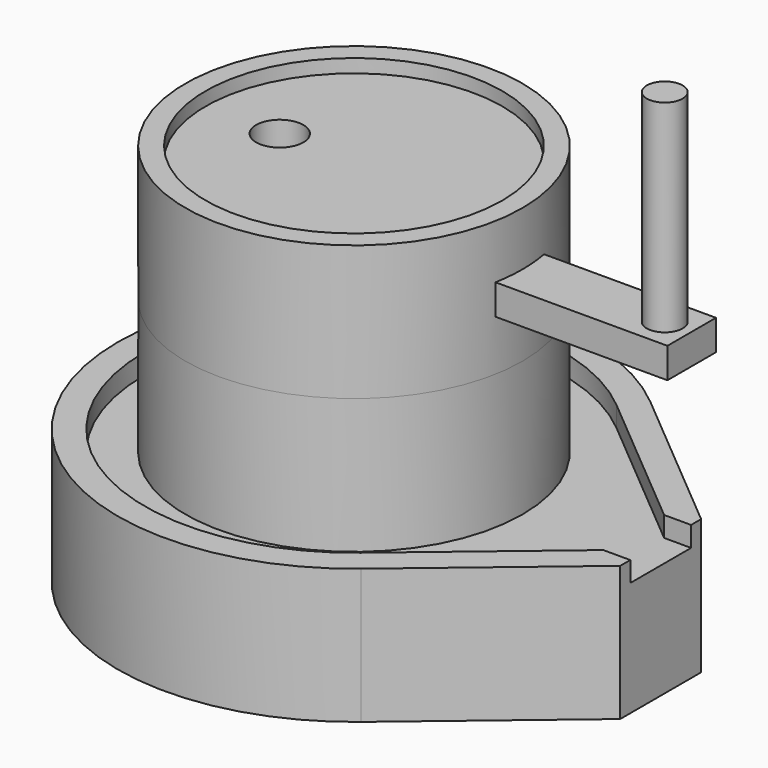
from build123d import *

# Parameters (mm, degrees)
F1_DEPTH  = 200
F3_DEPTH  = 30
F4_R      = 250
F5_DEPTH  = 200
F9_R      = 40
F10_DEPTH = 100
F11_R     = 250
F13_DEPTH = 200
F15_R     = 220
F16_DEPTH = 20
F17_R     = 35
F18_REACH = 648.9959493661
F21_DEPTH = 80
F22_W     = 90
F22_H     = 45
F23_DEPTH = 250
F24_R     = 15
F25_DEPTH = 30
F27_R     = 26.5702417315
F28_DEPTH = 300


with BuildPart() as f1:
    # F0 (on Top) → F1 (new body)
    with BuildSketch(Plane.XY):
        with BuildLine():
            ThreePointArc((225.1402542748, -267.977360807), (317.2531237011, -147.8189957411), (350, 0))
            ThreePointArc((350, 0), (317.2531237011, 147.8189957411), (225.1402542748, 267.977360807))
            ThreePointArc((225.1402542748, 267.977360807), (-350, 0), (225.1402542748, -267.977360807))
        make_face()
        with BuildLine():
            ThreePointArc((225.1402542748, 267.977360807), (317.2531237011, 147.8189957411), (350, 0))
            ThreePointArc((350, 0), (317.2531237011, -147.8189957411), (225.1402542748, -267.977360807))
            Line((225.1402542748, -267.977360807), (454.8351349665, -75))
            Line((454.8351349665, -75), (454.8351349665, 0))
            Line((454.8351349665, 0), (454.8351349665, 75))
            Line((454.8351349665, 75), (225.1402542748, 267.977360807))
        make_face()
    extrude(amount=F1_DEPTH)

    # F2 (on face) → F3 (cut)
    with BuildSketch(Plane.XY.offset(200)):
        with BuildLine():
            Line((414.8351349665, 56.3626426726), (199.4099395005, 237.3513767148))
            ThreePointArc((199.4099395005, 237.3513767148), (-310, 0), (199.4099395005, -237.3513767148))
            Line((199.4099395005, -237.3513767148), (414.8351349665, -56.3626426726))
            Line((414.8351349665, -56.3626426726), (454.8351349665, -56.3626426726))
            Line((454.8351349665, -56.3626426726), (454.8351349665, 56.3626426726))
            Line((454.8351349665, 56.3626426726), (414.8351349665, 56.3626426726))
        make_face()
    extrude(amount=-F3_DEPTH, mode=Mode.SUBTRACT)


with BuildPart() as f5:
    # F4 (on face) → F5 (new body)
    with BuildSketch(Plane.XY.offset(170)):
        Circle(F4_R)
    extrude(amount=F5_DEPTH)

    # F6 (on Front) → F7 (revolve)
    with BuildSketch(Plane.XZ):
        Polygon((0, 370), (0, 390), (-250, 370), align=None)
    revolve(axis=Axis((0, 0, 380), (0, 0, -1)))


with BuildPart() as f10:
    # F9 (on offset) → F10 (new body, symmetric)
    with BuildSketch(Plane.XY.offset(370)):
        Circle(F9_R)
    extrude(amount=F10_DEPTH, both=True)


with BuildPart() as f5_1:
    add(f5.part)

    # F12: cut F10
    add(f10.part, mode=Mode.SUBTRACT)


with BuildPart() as f13:
    # F11 (on offset) → F13 (new body)
    with BuildSketch(Plane.XY.offset(370)):
        Circle(F11_R)
    extrude(amount=F13_DEPTH)

    # F14: cut F10, F5
    add(f10.part, mode=Mode.SUBTRACT)
    add(f5_1.part, mode=Mode.SUBTRACT)

    # F15 (on face) → F16 (cut)
    with BuildSketch(Plane.XY.offset(570)):
        Circle(F15_R)
    extrude(amount=-F16_DEPTH, mode=Mode.SUBTRACT)

    f18_end = f5_1.part.faces().sort_by_distance((145, 0, 378.4))[0]
    # F17 (on face) → F18 (cut, up to a face of F5 that its end follows)
    with BuildSketch(Plane.XY.offset(550)):
        with Locations((-110, 0)):
            Circle(F17_R)
    f18_long = extrude(amount=-F18_REACH, mode=Mode.PRIVATE)
    add(split(f18_long, bisect_by=f18_end, keep=Keep.TOP, mode=Mode.PRIVATE), mode=Mode.SUBTRACT)


with BuildPart() as f21:
    # F20 (on offset) → F21 (new body)
    with BuildSketch(Plane.YZ.offset(250.8351349665)):
        Polygon((0, 490), (-45, 490), (-45, 445), (0, 445), (45, 445), (45, 490), align=None)
    extrude(amount=-F21_DEPTH)

    # F22 (on face) → F23 (join)
    with BuildSketch(Plane.YZ.offset(250.8351349665)):
        with Locations((0, 467.5)):
            Rectangle(F22_W, F22_H)
    extrude(amount=F23_DEPTH)


with BuildPart() as f25:
    # F24 (on face) → F25 (new body)
    with BuildSketch(Plane.XY.offset(490)):
        with Locations((460.8351349665, 0)):
            Circle(F24_R)
    extrude(amount=-F25_DEPTH)


with BuildPart() as f21_1:
    add(f21.part)

    # F26: cut F25
    add(f25.part, mode=Mode.SUBTRACT)


with BuildPart() as f25_1:
    add(f25.part)

    # F27 (on face) → F28 (join)
    with BuildSketch(Plane.XY.offset(490)):
        with Locations((460.8351349665, 0)):
            Circle(F27_R)
    extrude(amount=F28_DEPTH)


with BuildPart() as f13_1:
    add(f13.part)

    # F29: cut F21
    add(f21_1.part, mode=Mode.SUBTRACT)


solid = Compound([f1.part, f10.part, f5_1.part, f21_1.part, f25_1.part, f13_1.part])
